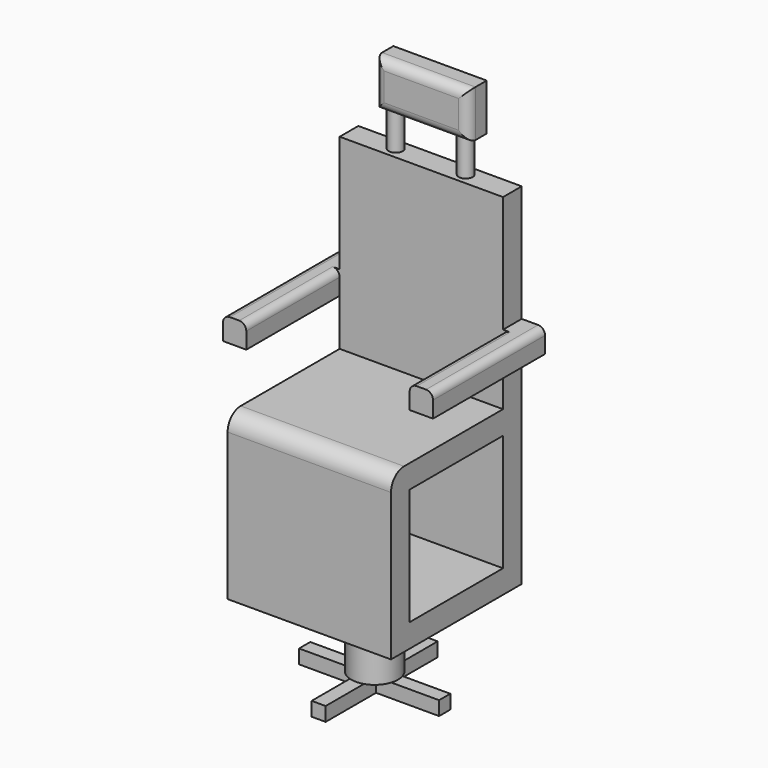
from build123d import *

# Parameters (mm, degrees)
F0_W          = 88.9
F0_H          = 88.9
F1_DEPTH      = 88.9
F2_W          = 63.5
F2_H          = 63.5
F3_DEPTH      = 88.9
F4_W          = 88.9
F4_H          = 12.7
F5_DEPTH      = 101.6
F6_R          = 12.7
F7_DEPTH      = 38.1
F8_W          = 7.62
F8_H          = 34.29
F8_H_2        = 7.62
F8_W_2        = 34.29
F9_DEPTH      = 7.62
F10_W         = 76.2
F10_H         = 12.7
F11_DEPTH     = 12.7
F12_W         = 76.2
F12_H         = 12.7
F13_DEPTH     = 12.7
F14_R         = 3.81
F15_DEPTH     = 19.05
F16_W         = 50.8
F16_H         = 12.7
F17_DEPTH     = 25.4
F18_R         = 8.89
F19_T1_DEPTH  = 76.2
F19_T3_DEPTH  = 50.8
F19_T8_DEPTH  = 76.2
F19_S9_R      = 3.81
F19_T10_DEPTH = 40
F19_S11_R     = 3.81
F19_T12_DEPTH = 40
F20_R         = 3.81


# Not quite as in the source:
# - a fillet or chamfer that OpenCascade refuses, or shapes differently, is made with other operations: its cross-section is extruded or revolved along the edge and cut away or added


with BuildPart() as f1:
    # F0 (on Top) → F1 (new body)
    with BuildSketch(Plane.XY):
        Rectangle(F0_W, F0_H)
    extrude(amount=F1_DEPTH)

    # F2 (on face) → F3 (cut)
    with BuildSketch(Plane.YZ.offset(44.45)):
        with Locations((0, 44.45)):
            Rectangle(F2_W, F2_H)
    extrude(amount=-F3_DEPTH, mode=Mode.SUBTRACT)

    # F4 (on face) → F5 (join)
    with BuildSketch(Plane.XY.offset(88.9)):
        with Locations((0, 38.1)):
            Rectangle(F4_W, F4_H)
    extrude(amount=F5_DEPTH)

    # F6 (on face) → F7 (join)
    with BuildSketch(Plane(origin=(0, 0, 0), x_dir=(1, 0, 0), z_dir=(0, 0, -1))):
        Circle(F6_R)
    extrude(amount=F7_DEPTH)

    # F8 (on face) → F9 (join)
    with BuildSketch(Plane(origin=(0, 0, -38.1), x_dir=(1, 0, 0), z_dir=(0, 0, -1))):
        with Locations((0, 20.955)):
            Rectangle(F8_W, F8_H)
        Rectangle(F8_W, F8_H_2)
        with Locations((-20.955, 0)):
            Rectangle(F8_W_2, F8_H_2)
        with Locations((20.955, 0)):
            Rectangle(F8_W_2, F8_H_2)
        with Locations((0, -20.955)):
            Rectangle(F8_W, F8_H)
    extrude(amount=F9_DEPTH)

    # F10 (on face) → F11 (join)
    with BuildSketch(Plane.YZ.offset(44.45)):
        with Locations((6.35, 120.65)):
            Rectangle(F10_W, F10_H)
    extrude(amount=F11_DEPTH)

    # F12 (on face) → F13 (join)
    with BuildSketch(Plane(origin=(-44.45, 0, 0), x_dir=(0, -1, 0), z_dir=(-1, 0, 0))):
        with Locations((-6.35, 120.65)):
            Rectangle(F12_W, F12_H)
    extrude(amount=F13_DEPTH)

    # F14 (on face) → F15 (join)
    with BuildSketch(Plane.XY.offset(190.5)):
        with Locations((19.05, 38.1)):
            Circle(F14_R)
        with Locations((-19.05, 38.1)):
            Circle(F14_R)
    extrude(amount=F15_DEPTH)

    # F16 (on face) → F17 (join)
    with BuildSketch(Plane.XY.offset(209.55)):
        with Locations((0, 38.1)):
            Rectangle(F16_W, F16_H)
    extrude(amount=F17_DEPTH)

    # F18
    f18_edges = [f1.edges().sort_by_distance(p)[0] for p in [
        (0, -44.45, 88.9),
    ]]
    fillet(f18_edges, radius=F18_R)

    # F19: fillet of radius 5.08 on 4 edges, made by hand

    # F19_s2 → F19_t1 (cut)
    with BuildSketch(Plane.YZ.offset(-38.1)):
        with BuildLine():
            ThreePointArc((31.75, 229.87), (33.2378975516, 233.4621024484), (36.83, 234.95))
            Line((36.83, 234.95), (31.75, 234.95))
            Line((31.75, 234.95), (31.75, 229.87))
        make_face()
    extrude(amount=F19_T1_DEPTH, mode=Mode.SUBTRACT)

    # F19_s4 → F19_t3 (cut)
    with BuildSketch(Plane.XY.offset(196.85)):
        with BuildLine():
            ThreePointArc((20.32, 31.75), (23.9121024484, 33.2378975516), (25.4, 36.83))
            Line((25.4, 36.83), (25.4, 31.75))
            Line((25.4, 31.75), (20.32, 31.75))
        make_face()
        with BuildLine():
            ThreePointArc((-20.32, 31.75), (-23.9121024484, 33.2378975516), (-25.4, 36.83))
            Line((-25.4, 36.83), (-25.4, 31.75))
            Line((-25.4, 31.75), (-20.32, 31.75))
        make_face()
    extrude(amount=F19_T3_DEPTH, mode=Mode.SUBTRACT)


with BuildPart() as f19_tool6:
    # F19_s7 → F19_t8 (new body)
    with BuildSketch(Plane.YZ.offset(-38.1)):
        with BuildLine():
            ThreePointArc((36.83, 209.55), (33.2378975516, 211.0378975516), (31.75, 214.63))
            Line((31.75, 214.63), (31.75, 209.55))
            Line((31.75, 209.55), (36.83, 209.55))
        make_face()
    extrude(amount=F19_T8_DEPTH)

    # F19_s9 → F19_t10 (cut, symmetric)
    with BuildSketch(Plane.XY.offset(212.1)):
        with Locations((-19.05, 38.1)):
            Circle(F19_S9_R)
    extrude(amount=F19_T10_DEPTH, both=True, mode=Mode.SUBTRACT)

    # F19_s11 → F19_t12 (cut, symmetric)
    with BuildSketch(Plane.XY.offset(212.1)):
        with Locations((19.05, 38.1)):
            Circle(F19_S11_R)
    extrude(amount=F19_T12_DEPTH, both=True, mode=Mode.SUBTRACT)


with BuildPart() as f1_1:
    add(f1.part)

    # F19_t5: cut F19_tool6
    add(f19_tool6.part, mode=Mode.SUBTRACT)

    # F20
    f20_edges = [f1_1.edges().sort_by_distance(p)[0] for p in [
        (44.45, 0, 127),
        (57.15, 6.35, 127),
        (-44.45, 0, 127),
        (-57.15, 6.35, 127),
    ]]
    fillet(f20_edges, radius=F20_R)


solid = f1_1.part
